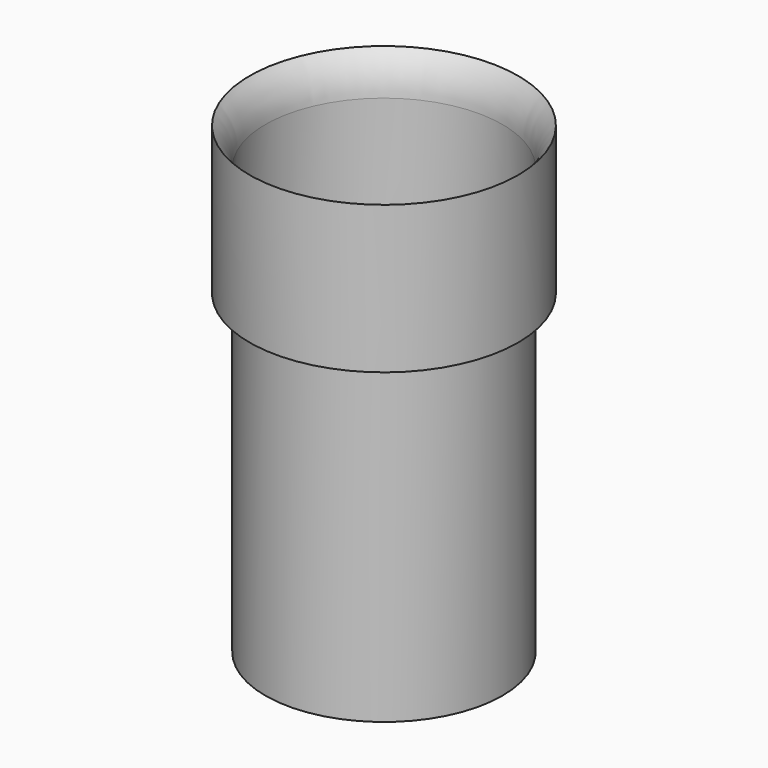
from build123d import *

# Parameters (mm, degrees)
F0_R     = 12.75
F0_R_2   = 11.25
F1_DEPTH = 14
F2_R     = 11.25
F2_R_2   = 10
F3_DEPTH = 30


# Not quite as in the source:
# - a fillet or chamfer that OpenCascade refuses, or shapes differently, is made with other operations: its cross-section is extruded or revolved along the edge and cut away or added


with BuildPart() as f1:
    # F0 (on Top) → F1 (new body)
    with BuildSketch(Plane.XY):
        Circle(F0_R)
        Circle(F0_R_2, mode=Mode.SUBTRACT)
    extrude(amount=F1_DEPTH)

    # F5: fillet of radius 5 on 1 edges, made by hand

    # F5_s1 → F5_t2 (revolve, cut)
    with BuildSketch(Plane.XZ):
        with BuildLine():
            ThreePointArc((11.25, 10.4292857857), (11.6402277714, 12.3657774588), (12.75, 14))
            Line((12.75, 14), (11.25, 14))
            Line((11.25, 14), (11.25, 10.4292857857))
        make_face()
    revolve(axis=Axis((0, 0, 14), (0, 0, 1)), mode=Mode.SUBTRACT)


with BuildPart() as f3:
    # F2 (on Top) → F3 (new body)
    with BuildSketch(Plane.XY):
        Circle(F2_R)
        Circle(F2_R_2, mode=Mode.SUBTRACT)
    extrude(amount=-F3_DEPTH)

    # F4: fillet of radius 10 on 1 edges, made by hand

    # F4_s1 → F4_t2 (revolve, cut)
    with BuildSketch(Plane.XZ):
        with BuildLine():
            add(Edge.make_bspline(
                [(10, -4.8412291828), (10, -2.2592402853), (11.25, 0)],
                knots=[0, 0, 0, 1, 1, 1], degree=2, weights=[1, 0.1111111111, 1]))
            Line((11.25, 0), (10, 0))
            Line((10, 0), (10, -4.8412291828))
        make_face()
    revolve(axis=Axis((0, 0, 0), (0, 0, 1)), mode=Mode.SUBTRACT)

    # F6: fillet of radius 5 on 1 edges, made by hand

    # F6_s1 → F6_t2 (revolve, cut)
    with BuildSketch(Plane.XZ):
        with BuildLine():
            ThreePointArc((11.25, -30), (10.3229282665, -28.4605778141), (10, -26.6928108612))
            Line((10, -26.6928108612), (10, -30))
            Line((10, -30), (11.25, -30))
        make_face()
    revolve(axis=Axis((0, 0, -30), (0, 0, 1)), mode=Mode.SUBTRACT)


solid = Compound([f1.part, f3.part])
